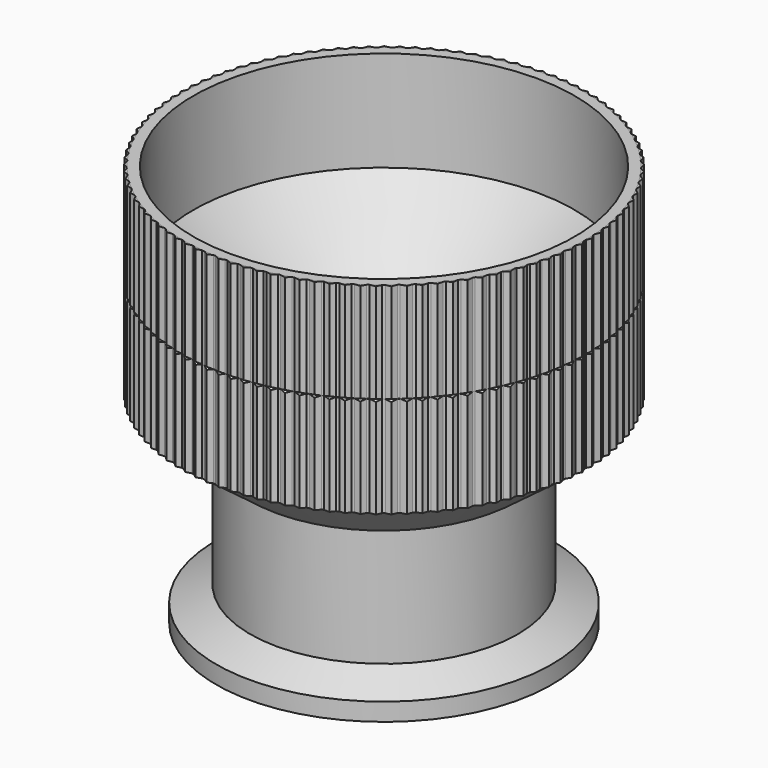
from build123d import *

# Parameters (mm, degrees)
F0_R      = 6
F1_DEPTH  = 6
F2_R      = 5.6
F3_DEPTH  = 3
F10_DEPTH = 31
F11_DEPTH = 25
F12_COUNT = 105


with BuildPart() as f1:
    # F0 (on Right) → F1 (new body)
    with BuildSketch(Plane.YZ):
        Circle(F0_R)
    extrude(amount=F1_DEPTH)

    # F2 (on face) → F3 (cut)
    with BuildSketch(Plane.YZ.offset(6)):
        Circle(F2_R)
    extrude(amount=-F3_DEPTH, mode=Mode.SUBTRACT)


with BuildPart() as f6:
    # F5 (on Right) → F6 (revolve)
    with BuildSketch(Plane.YZ):
        Polygon((6, 4.305355005), (6, 10.305355005), (5.6948992424, 10.305355005), (5.6948992424, 7.305355005), (3.011390429, 4.305355005), (3.011390429, 2.805355005), (3.011390429, -1.694644995), (5.011390429, -1.694644995), (5.011390429, -1.4897467336), (5.011390429, -1.1619703146), (4, -0.694644995), (4, 2.805355005), align=None)
    revolve(axis=Axis((0, 0, 5.6095318998), (0, 0, -1)))


with BuildPart() as f10:
    # F9 (on offset) → F10 (new body)
    with BuildSketch(Plane.XY.offset(35.305355005)):
        Polygon((-5.9907040559, -0.15034221), (-5.9907040559, 0.1501146035), (-6.068165414, 0), align=None)
    extrude(amount=-F10_DEPTH)

    # F11 (cut): a face of the model
    f11_faces = [f10.faces().sort_by_distance(p)[0] for p in [
        (-6.0165245086, -7.58688e-05, 35.305355005),
    ]]
    extrude(f11_faces, amount=-F11_DEPTH, mode=Mode.SUBTRACT)


with BuildPart() as f12_1:
    # F12: instance of F10
    add(f10.part.rotate(Axis((0, 0, 4.305355005), (0, 0, -1)), 1 * 360 / F12_COUNT))


with BuildPart() as f12_2:
    # F12: instance of F10
    add(f10.part.rotate(Axis((0, 0, 4.305355005), (0, 0, -1)), 2 * 360 / F12_COUNT))


with BuildPart() as f12_3:
    # F12: instance of F10
    add(f10.part.rotate(Axis((0, 0, 4.305355005), (0, 0, -1)), 3 * 360 / F12_COUNT))


with BuildPart() as f12_4:
    # F12: instance of F10
    add(f10.part.rotate(Axis((0, 0, 4.305355005), (0, 0, -1)), 4 * 360 / F12_COUNT))


with BuildPart() as f12_5:
    # F12: instance of F10
    add(f10.part.rotate(Axis((0, 0, 4.305355005), (0, 0, -1)), 5 * 360 / F12_COUNT))


with BuildPart() as f12_6:
    # F12: instance of F10
    add(f10.part.rotate(Axis((0, 0, 4.305355005), (0, 0, -1)), 6 * 360 / F12_COUNT))


with BuildPart() as f12_7:
    # F12: instance of F10
    add(f10.part.rotate(Axis((0, 0, 4.305355005), (0, 0, -1)), 7 * 360 / F12_COUNT))


with BuildPart() as f12_8:
    # F12: instance of F10
    add(f10.part.rotate(Axis((0, 0, 4.305355005), (0, 0, -1)), 8 * 360 / F12_COUNT))


with BuildPart() as f12_9:
    # F12: instance of F10
    add(f10.part.rotate(Axis((0, 0, 4.305355005), (0, 0, -1)), 9 * 360 / F12_COUNT))


with BuildPart() as f12_10:
    # F12: instance of F10
    add(f10.part.rotate(Axis((0, 0, 4.305355005), (0, 0, -1)), 10 * 360 / F12_COUNT))


with BuildPart() as f12_11:
    # F12: instance of F10
    add(f10.part.rotate(Axis((0, 0, 4.305355005), (0, 0, -1)), 11 * 360 / F12_COUNT))


with BuildPart() as f12_12:
    # F12: instance of F10
    add(f10.part.rotate(Axis((0, 0, 4.305355005), (0, 0, -1)), 12 * 360 / F12_COUNT))


with BuildPart() as f12_13:
    # F12: instance of F10
    add(f10.part.rotate(Axis((0, 0, 4.305355005), (0, 0, -1)), 13 * 360 / F12_COUNT))


with BuildPart() as f12_14:
    # F12: instance of F10
    add(f10.part.rotate(Axis((0, 0, 4.305355005), (0, 0, -1)), 14 * 360 / F12_COUNT))


with BuildPart() as f12_15:
    # F12: instance of F10
    add(f10.part.rotate(Axis((0, 0, 4.305355005), (0, 0, -1)), 15 * 360 / F12_COUNT))


with BuildPart() as f12_16:
    # F12: instance of F10
    add(f10.part.rotate(Axis((0, 0, 4.305355005), (0, 0, -1)), 16 * 360 / F12_COUNT))


with BuildPart() as f12_17:
    # F12: instance of F10
    add(f10.part.rotate(Axis((0, 0, 4.305355005), (0, 0, -1)), 17 * 360 / F12_COUNT))


with BuildPart() as f12_18:
    # F12: instance of F10
    add(f10.part.rotate(Axis((0, 0, 4.305355005), (0, 0, -1)), 18 * 360 / F12_COUNT))


with BuildPart() as f12_19:
    # F12: instance of F10
    add(f10.part.rotate(Axis((0, 0, 4.305355005), (0, 0, -1)), 19 * 360 / F12_COUNT))


with BuildPart() as f12_20:
    # F12: instance of F10
    add(f10.part.rotate(Axis((0, 0, 4.305355005), (0, 0, -1)), 20 * 360 / F12_COUNT))


with BuildPart() as f12_21:
    # F12: instance of F10
    add(f10.part.rotate(Axis((0, 0, 4.305355005), (0, 0, -1)), 21 * 360 / F12_COUNT))


with BuildPart() as f12_22:
    # F12: instance of F10
    add(f10.part.rotate(Axis((0, 0, 4.305355005), (0, 0, -1)), 22 * 360 / F12_COUNT))


with BuildPart() as f12_23:
    # F12: instance of F10
    add(f10.part.rotate(Axis((0, 0, 4.305355005), (0, 0, -1)), 23 * 360 / F12_COUNT))


with BuildPart() as f12_24:
    # F12: instance of F10
    add(f10.part.rotate(Axis((0, 0, 4.305355005), (0, 0, -1)), 24 * 360 / F12_COUNT))


with BuildPart() as f12_25:
    # F12: instance of F10
    add(f10.part.rotate(Axis((0, 0, 4.305355005), (0, 0, -1)), 25 * 360 / F12_COUNT))


with BuildPart() as f12_26:
    # F12: instance of F10
    add(f10.part.rotate(Axis((0, 0, 4.305355005), (0, 0, -1)), 26 * 360 / F12_COUNT))


with BuildPart() as f12_27:
    # F12: instance of F10
    add(f10.part.rotate(Axis((0, 0, 4.305355005), (0, 0, -1)), 27 * 360 / F12_COUNT))


with BuildPart() as f12_28:
    # F12: instance of F10
    add(f10.part.rotate(Axis((0, 0, 4.305355005), (0, 0, -1)), 28 * 360 / F12_COUNT))


with BuildPart() as f12_29:
    # F12: instance of F10
    add(f10.part.rotate(Axis((0, 0, 4.305355005), (0, 0, -1)), 29 * 360 / F12_COUNT))


with BuildPart() as f12_30:
    # F12: instance of F10
    add(f10.part.rotate(Axis((0, 0, 4.305355005), (0, 0, -1)), 30 * 360 / F12_COUNT))


with BuildPart() as f12_31:
    # F12: instance of F10
    add(f10.part.rotate(Axis((0, 0, 4.305355005), (0, 0, -1)), 31 * 360 / F12_COUNT))


with BuildPart() as f12_32:
    # F12: instance of F10
    add(f10.part.rotate(Axis((0, 0, 4.305355005), (0, 0, -1)), 32 * 360 / F12_COUNT))


with BuildPart() as f12_33:
    # F12: instance of F10
    add(f10.part.rotate(Axis((0, 0, 4.305355005), (0, 0, -1)), 33 * 360 / F12_COUNT))


with BuildPart() as f12_34:
    # F12: instance of F10
    add(f10.part.rotate(Axis((0, 0, 4.305355005), (0, 0, -1)), 34 * 360 / F12_COUNT))


with BuildPart() as f12_35:
    # F12: instance of F10
    add(f10.part.rotate(Axis((0, 0, 4.305355005), (0, 0, -1)), 35 * 360 / F12_COUNT))


with BuildPart() as f12_36:
    # F12: instance of F10
    add(f10.part.rotate(Axis((0, 0, 4.305355005), (0, 0, -1)), 36 * 360 / F12_COUNT))


with BuildPart() as f12_37:
    # F12: instance of F10
    add(f10.part.rotate(Axis((0, 0, 4.305355005), (0, 0, -1)), 37 * 360 / F12_COUNT))


with BuildPart() as f12_38:
    # F12: instance of F10
    add(f10.part.rotate(Axis((0, 0, 4.305355005), (0, 0, -1)), 38 * 360 / F12_COUNT))


with BuildPart() as f12_39:
    # F12: instance of F10
    add(f10.part.rotate(Axis((0, 0, 4.305355005), (0, 0, -1)), 39 * 360 / F12_COUNT))


with BuildPart() as f12_40:
    # F12: instance of F10
    add(f10.part.rotate(Axis((0, 0, 4.305355005), (0, 0, -1)), 40 * 360 / F12_COUNT))


with BuildPart() as f12_41:
    # F12: instance of F10
    add(f10.part.rotate(Axis((0, 0, 4.305355005), (0, 0, -1)), 41 * 360 / F12_COUNT))


with BuildPart() as f12_42:
    # F12: instance of F10
    add(f10.part.rotate(Axis((0, 0, 4.305355005), (0, 0, -1)), 42 * 360 / F12_COUNT))


with BuildPart() as f12_43:
    # F12: instance of F10
    add(f10.part.rotate(Axis((0, 0, 4.305355005), (0, 0, -1)), 43 * 360 / F12_COUNT))


with BuildPart() as f12_44:
    # F12: instance of F10
    add(f10.part.rotate(Axis((0, 0, 4.305355005), (0, 0, -1)), 44 * 360 / F12_COUNT))


with BuildPart() as f12_45:
    # F12: instance of F10
    add(f10.part.rotate(Axis((0, 0, 4.305355005), (0, 0, -1)), 45 * 360 / F12_COUNT))


with BuildPart() as f12_46:
    # F12: instance of F10
    add(f10.part.rotate(Axis((0, 0, 4.305355005), (0, 0, -1)), 46 * 360 / F12_COUNT))


with BuildPart() as f12_47:
    # F12: instance of F10
    add(f10.part.rotate(Axis((0, 0, 4.305355005), (0, 0, -1)), 47 * 360 / F12_COUNT))


with BuildPart() as f12_48:
    # F12: instance of F10
    add(f10.part.rotate(Axis((0, 0, 4.305355005), (0, 0, -1)), 48 * 360 / F12_COUNT))


with BuildPart() as f12_49:
    # F12: instance of F10
    add(f10.part.rotate(Axis((0, 0, 4.305355005), (0, 0, -1)), 49 * 360 / F12_COUNT))


with BuildPart() as f12_50:
    # F12: instance of F10
    add(f10.part.rotate(Axis((0, 0, 4.305355005), (0, 0, -1)), 50 * 360 / F12_COUNT))


with BuildPart() as f12_51:
    # F12: instance of F10
    add(f10.part.rotate(Axis((0, 0, 4.305355005), (0, 0, -1)), 51 * 360 / F12_COUNT))


with BuildPart() as f12_52:
    # F12: instance of F10
    add(f10.part.rotate(Axis((0, 0, 4.305355005), (0, 0, -1)), 52 * 360 / F12_COUNT))


with BuildPart() as f12_53:
    # F12: instance of F10
    add(f10.part.rotate(Axis((0, 0, 4.305355005), (0, 0, -1)), 53 * 360 / F12_COUNT))


with BuildPart() as f12_54:
    # F12: instance of F10
    add(f10.part.rotate(Axis((0, 0, 4.305355005), (0, 0, -1)), 54 * 360 / F12_COUNT))


with BuildPart() as f12_55:
    # F12: instance of F10
    add(f10.part.rotate(Axis((0, 0, 4.305355005), (0, 0, -1)), 55 * 360 / F12_COUNT))


with BuildPart() as f12_56:
    # F12: instance of F10
    add(f10.part.rotate(Axis((0, 0, 4.305355005), (0, 0, -1)), 56 * 360 / F12_COUNT))


with BuildPart() as f12_57:
    # F12: instance of F10
    add(f10.part.rotate(Axis((0, 0, 4.305355005), (0, 0, -1)), 57 * 360 / F12_COUNT))


with BuildPart() as f12_58:
    # F12: instance of F10
    add(f10.part.rotate(Axis((0, 0, 4.305355005), (0, 0, -1)), 58 * 360 / F12_COUNT))


with BuildPart() as f12_59:
    # F12: instance of F10
    add(f10.part.rotate(Axis((0, 0, 4.305355005), (0, 0, -1)), 59 * 360 / F12_COUNT))


with BuildPart() as f12_60:
    # F12: instance of F10
    add(f10.part.rotate(Axis((0, 0, 4.305355005), (0, 0, -1)), 60 * 360 / F12_COUNT))


with BuildPart() as f12_61:
    # F12: instance of F10
    add(f10.part.rotate(Axis((0, 0, 4.305355005), (0, 0, -1)), 61 * 360 / F12_COUNT))


with BuildPart() as f12_62:
    # F12: instance of F10
    add(f10.part.rotate(Axis((0, 0, 4.305355005), (0, 0, -1)), 62 * 360 / F12_COUNT))


with BuildPart() as f12_63:
    # F12: instance of F10
    add(f10.part.rotate(Axis((0, 0, 4.305355005), (0, 0, -1)), 63 * 360 / F12_COUNT))


with BuildPart() as f12_64:
    # F12: instance of F10
    add(f10.part.rotate(Axis((0, 0, 4.305355005), (0, 0, -1)), 64 * 360 / F12_COUNT))


with BuildPart() as f12_65:
    # F12: instance of F10
    add(f10.part.rotate(Axis((0, 0, 4.305355005), (0, 0, -1)), 65 * 360 / F12_COUNT))


with BuildPart() as f12_66:
    # F12: instance of F10
    add(f10.part.rotate(Axis((0, 0, 4.305355005), (0, 0, -1)), 66 * 360 / F12_COUNT))


with BuildPart() as f12_67:
    # F12: instance of F10
    add(f10.part.rotate(Axis((0, 0, 4.305355005), (0, 0, -1)), 67 * 360 / F12_COUNT))


with BuildPart() as f12_68:
    # F12: instance of F10
    add(f10.part.rotate(Axis((0, 0, 4.305355005), (0, 0, -1)), 68 * 360 / F12_COUNT))


with BuildPart() as f12_69:
    # F12: instance of F10
    add(f10.part.rotate(Axis((0, 0, 4.305355005), (0, 0, -1)), 69 * 360 / F12_COUNT))


with BuildPart() as f12_70:
    # F12: instance of F10
    add(f10.part.rotate(Axis((0, 0, 4.305355005), (0, 0, -1)), 70 * 360 / F12_COUNT))


with BuildPart() as f12_71:
    # F12: instance of F10
    add(f10.part.rotate(Axis((0, 0, 4.305355005), (0, 0, -1)), 71 * 360 / F12_COUNT))


with BuildPart() as f12_72:
    # F12: instance of F10
    add(f10.part.rotate(Axis((0, 0, 4.305355005), (0, 0, -1)), 72 * 360 / F12_COUNT))


with BuildPart() as f12_73:
    # F12: instance of F10
    add(f10.part.rotate(Axis((0, 0, 4.305355005), (0, 0, -1)), 73 * 360 / F12_COUNT))


with BuildPart() as f12_74:
    # F12: instance of F10
    add(f10.part.rotate(Axis((0, 0, 4.305355005), (0, 0, -1)), 74 * 360 / F12_COUNT))


with BuildPart() as f12_75:
    # F12: instance of F10
    add(f10.part.rotate(Axis((0, 0, 4.305355005), (0, 0, -1)), 75 * 360 / F12_COUNT))


with BuildPart() as f12_76:
    # F12: instance of F10
    add(f10.part.rotate(Axis((0, 0, 4.305355005), (0, 0, -1)), 76 * 360 / F12_COUNT))


with BuildPart() as f12_77:
    # F12: instance of F10
    add(f10.part.rotate(Axis((0, 0, 4.305355005), (0, 0, -1)), 77 * 360 / F12_COUNT))


with BuildPart() as f12_78:
    # F12: instance of F10
    add(f10.part.rotate(Axis((0, 0, 4.305355005), (0, 0, -1)), 78 * 360 / F12_COUNT))


with BuildPart() as f12_79:
    # F12: instance of F10
    add(f10.part.rotate(Axis((0, 0, 4.305355005), (0, 0, -1)), 79 * 360 / F12_COUNT))


with BuildPart() as f12_80:
    # F12: instance of F10
    add(f10.part.rotate(Axis((0, 0, 4.305355005), (0, 0, -1)), 80 * 360 / F12_COUNT))


with BuildPart() as f12_81:
    # F12: instance of F10
    add(f10.part.rotate(Axis((0, 0, 4.305355005), (0, 0, -1)), 81 * 360 / F12_COUNT))


with BuildPart() as f12_82:
    # F12: instance of F10
    add(f10.part.rotate(Axis((0, 0, 4.305355005), (0, 0, -1)), 82 * 360 / F12_COUNT))


with BuildPart() as f12_83:
    # F12: instance of F10
    add(f10.part.rotate(Axis((0, 0, 4.305355005), (0, 0, -1)), 83 * 360 / F12_COUNT))


with BuildPart() as f12_84:
    # F12: instance of F10
    add(f10.part.rotate(Axis((0, 0, 4.305355005), (0, 0, -1)), 84 * 360 / F12_COUNT))


with BuildPart() as f12_85:
    # F12: instance of F10
    add(f10.part.rotate(Axis((0, 0, 4.305355005), (0, 0, -1)), 85 * 360 / F12_COUNT))


with BuildPart() as f12_86:
    # F12: instance of F10
    add(f10.part.rotate(Axis((0, 0, 4.305355005), (0, 0, -1)), 86 * 360 / F12_COUNT))


with BuildPart() as f12_87:
    # F12: instance of F10
    add(f10.part.rotate(Axis((0, 0, 4.305355005), (0, 0, -1)), 87 * 360 / F12_COUNT))


with BuildPart() as f12_88:
    # F12: instance of F10
    add(f10.part.rotate(Axis((0, 0, 4.305355005), (0, 0, -1)), 88 * 360 / F12_COUNT))


with BuildPart() as f12_89:
    # F12: instance of F10
    add(f10.part.rotate(Axis((0, 0, 4.305355005), (0, 0, -1)), 89 * 360 / F12_COUNT))


with BuildPart() as f12_90:
    # F12: instance of F10
    add(f10.part.rotate(Axis((0, 0, 4.305355005), (0, 0, -1)), 90 * 360 / F12_COUNT))


with BuildPart() as f12_91:
    # F12: instance of F10
    add(f10.part.rotate(Axis((0, 0, 4.305355005), (0, 0, -1)), 91 * 360 / F12_COUNT))


with BuildPart() as f12_92:
    # F12: instance of F10
    add(f10.part.rotate(Axis((0, 0, 4.305355005), (0, 0, -1)), 92 * 360 / F12_COUNT))


with BuildPart() as f12_93:
    # F12: instance of F10
    add(f10.part.rotate(Axis((0, 0, 4.305355005), (0, 0, -1)), 93 * 360 / F12_COUNT))


with BuildPart() as f12_94:
    # F12: instance of F10
    add(f10.part.rotate(Axis((0, 0, 4.305355005), (0, 0, -1)), 94 * 360 / F12_COUNT))


with BuildPart() as f12_95:
    # F12: instance of F10
    add(f10.part.rotate(Axis((0, 0, 4.305355005), (0, 0, -1)), 95 * 360 / F12_COUNT))


with BuildPart() as f12_96:
    # F12: instance of F10
    add(f10.part.rotate(Axis((0, 0, 4.305355005), (0, 0, -1)), 96 * 360 / F12_COUNT))


with BuildPart() as f12_97:
    # F12: instance of F10
    add(f10.part.rotate(Axis((0, 0, 4.305355005), (0, 0, -1)), 97 * 360 / F12_COUNT))


with BuildPart() as f12_98:
    # F12: instance of F10
    add(f10.part.rotate(Axis((0, 0, 4.305355005), (0, 0, -1)), 98 * 360 / F12_COUNT))


with BuildPart() as f12_99:
    # F12: instance of F10
    add(f10.part.rotate(Axis((0, 0, 4.305355005), (0, 0, -1)), 99 * 360 / F12_COUNT))


with BuildPart() as f12_100:
    # F12: instance of F10
    add(f10.part.rotate(Axis((0, 0, 4.305355005), (0, 0, -1)), 100 * 360 / F12_COUNT))


with BuildPart() as f12_101:
    # F12: instance of F10
    add(f10.part.rotate(Axis((0, 0, 4.305355005), (0, 0, -1)), 101 * 360 / F12_COUNT))


with BuildPart() as f12_102:
    # F12: instance of F10
    add(f10.part.rotate(Axis((0, 0, 4.305355005), (0, 0, -1)), 102 * 360 / F12_COUNT))


with BuildPart() as f12_103:
    # F12: instance of F10
    add(f10.part.rotate(Axis((0, 0, 4.305355005), (0, 0, -1)), 103 * 360 / F12_COUNT))


with BuildPart() as f12_104:
    # F12: instance of F10
    add(f10.part.rotate(Axis((0, 0, 4.305355005), (0, 0, -1)), 104 * 360 / F12_COUNT))


with BuildPart() as f14_tool:
    # F13 (on Front) → F14 (revolve)
    with BuildSketch(Plane.XZ):
        Polygon((6.091067441, 7.3605600495), (5.9954494991, 7.305355005), (6.091067441, 7.2501499605), align=None)
    revolve(axis=Axis((0, 0, 6.7933266461), (0, 0, -1)))


with BuildPart() as f6_1:
    add(f6.part)

    # F14: cut by f14_tool
    add(f14_tool.part, mode=Mode.SUBTRACT)


with BuildPart() as f10_1:
    add(f10.part)

    # F14: cut by f14_tool
    add(f14_tool.part, mode=Mode.SUBTRACT)


with BuildPart() as f12_1_1:
    add(f12_1.part)

    # F14: cut by f14_tool
    add(f14_tool.part, mode=Mode.SUBTRACT)


with BuildPart() as f12_2_1:
    add(f12_2.part)

    # F14: cut by f14_tool
    add(f14_tool.part, mode=Mode.SUBTRACT)


with BuildPart() as f12_3_1:
    add(f12_3.part)

    # F14: cut by f14_tool
    add(f14_tool.part, mode=Mode.SUBTRACT)


with BuildPart() as f12_4_1:
    add(f12_4.part)

    # F14: cut by f14_tool
    add(f14_tool.part, mode=Mode.SUBTRACT)


with BuildPart() as f12_5_1:
    add(f12_5.part)

    # F14: cut by f14_tool
    add(f14_tool.part, mode=Mode.SUBTRACT)


with BuildPart() as f12_6_1:
    add(f12_6.part)

    # F14: cut by f14_tool
    add(f14_tool.part, mode=Mode.SUBTRACT)


with BuildPart() as f12_7_1:
    add(f12_7.part)

    # F14: cut by f14_tool
    add(f14_tool.part, mode=Mode.SUBTRACT)


with BuildPart() as f12_8_1:
    add(f12_8.part)

    # F14: cut by f14_tool
    add(f14_tool.part, mode=Mode.SUBTRACT)


with BuildPart() as f12_9_1:
    add(f12_9.part)

    # F14: cut by f14_tool
    add(f14_tool.part, mode=Mode.SUBTRACT)


with BuildPart() as f12_10_1:
    add(f12_10.part)

    # F14: cut by f14_tool
    add(f14_tool.part, mode=Mode.SUBTRACT)


with BuildPart() as f12_11_1:
    add(f12_11.part)

    # F14: cut by f14_tool
    add(f14_tool.part, mode=Mode.SUBTRACT)


with BuildPart() as f12_12_1:
    add(f12_12.part)

    # F14: cut by f14_tool
    add(f14_tool.part, mode=Mode.SUBTRACT)


with BuildPart() as f12_13_1:
    add(f12_13.part)

    # F14: cut by f14_tool
    add(f14_tool.part, mode=Mode.SUBTRACT)


with BuildPart() as f12_14_1:
    add(f12_14.part)

    # F14: cut by f14_tool
    add(f14_tool.part, mode=Mode.SUBTRACT)


with BuildPart() as f12_15_1:
    add(f12_15.part)

    # F14: cut by f14_tool
    add(f14_tool.part, mode=Mode.SUBTRACT)


with BuildPart() as f12_16_1:
    add(f12_16.part)

    # F14: cut by f14_tool
    add(f14_tool.part, mode=Mode.SUBTRACT)


with BuildPart() as f12_17_1:
    add(f12_17.part)

    # F14: cut by f14_tool
    add(f14_tool.part, mode=Mode.SUBTRACT)


with BuildPart() as f12_18_1:
    add(f12_18.part)

    # F14: cut by f14_tool
    add(f14_tool.part, mode=Mode.SUBTRACT)


with BuildPart() as f12_19_1:
    add(f12_19.part)

    # F14: cut by f14_tool
    add(f14_tool.part, mode=Mode.SUBTRACT)


with BuildPart() as f12_20_1:
    add(f12_20.part)

    # F14: cut by f14_tool
    add(f14_tool.part, mode=Mode.SUBTRACT)


with BuildPart() as f12_21_1:
    add(f12_21.part)

    # F14: cut by f14_tool
    add(f14_tool.part, mode=Mode.SUBTRACT)


with BuildPart() as f12_22_1:
    add(f12_22.part)

    # F14: cut by f14_tool
    add(f14_tool.part, mode=Mode.SUBTRACT)


with BuildPart() as f12_23_1:
    add(f12_23.part)

    # F14: cut by f14_tool
    add(f14_tool.part, mode=Mode.SUBTRACT)


with BuildPart() as f12_24_1:
    add(f12_24.part)

    # F14: cut by f14_tool
    add(f14_tool.part, mode=Mode.SUBTRACT)


with BuildPart() as f12_25_1:
    add(f12_25.part)

    # F14: cut by f14_tool
    add(f14_tool.part, mode=Mode.SUBTRACT)


with BuildPart() as f12_26_1:
    add(f12_26.part)

    # F14: cut by f14_tool
    add(f14_tool.part, mode=Mode.SUBTRACT)


with BuildPart() as f12_27_1:
    add(f12_27.part)

    # F14: cut by f14_tool
    add(f14_tool.part, mode=Mode.SUBTRACT)


with BuildPart() as f12_28_1:
    add(f12_28.part)

    # F14: cut by f14_tool
    add(f14_tool.part, mode=Mode.SUBTRACT)


with BuildPart() as f12_29_1:
    add(f12_29.part)

    # F14: cut by f14_tool
    add(f14_tool.part, mode=Mode.SUBTRACT)


with BuildPart() as f12_30_1:
    add(f12_30.part)

    # F14: cut by f14_tool
    add(f14_tool.part, mode=Mode.SUBTRACT)


with BuildPart() as f12_31_1:
    add(f12_31.part)

    # F14: cut by f14_tool
    add(f14_tool.part, mode=Mode.SUBTRACT)


with BuildPart() as f12_32_1:
    add(f12_32.part)

    # F14: cut by f14_tool
    add(f14_tool.part, mode=Mode.SUBTRACT)


with BuildPart() as f12_33_1:
    add(f12_33.part)

    # F14: cut by f14_tool
    add(f14_tool.part, mode=Mode.SUBTRACT)


with BuildPart() as f12_34_1:
    add(f12_34.part)

    # F14: cut by f14_tool
    add(f14_tool.part, mode=Mode.SUBTRACT)


with BuildPart() as f12_35_1:
    add(f12_35.part)

    # F14: cut by f14_tool
    add(f14_tool.part, mode=Mode.SUBTRACT)


with BuildPart() as f12_36_1:
    add(f12_36.part)

    # F14: cut by f14_tool
    add(f14_tool.part, mode=Mode.SUBTRACT)


with BuildPart() as f12_37_1:
    add(f12_37.part)

    # F14: cut by f14_tool
    add(f14_tool.part, mode=Mode.SUBTRACT)


with BuildPart() as f12_38_1:
    add(f12_38.part)

    # F14: cut by f14_tool
    add(f14_tool.part, mode=Mode.SUBTRACT)


with BuildPart() as f12_39_1:
    add(f12_39.part)

    # F14: cut by f14_tool
    add(f14_tool.part, mode=Mode.SUBTRACT)


with BuildPart() as f12_40_1:
    add(f12_40.part)

    # F14: cut by f14_tool
    add(f14_tool.part, mode=Mode.SUBTRACT)


with BuildPart() as f12_41_1:
    add(f12_41.part)

    # F14: cut by f14_tool
    add(f14_tool.part, mode=Mode.SUBTRACT)


with BuildPart() as f12_42_1:
    add(f12_42.part)

    # F14: cut by f14_tool
    add(f14_tool.part, mode=Mode.SUBTRACT)


with BuildPart() as f12_43_1:
    add(f12_43.part)

    # F14: cut by f14_tool
    add(f14_tool.part, mode=Mode.SUBTRACT)


with BuildPart() as f12_44_1:
    add(f12_44.part)

    # F14: cut by f14_tool
    add(f14_tool.part, mode=Mode.SUBTRACT)


with BuildPart() as f12_45_1:
    add(f12_45.part)

    # F14: cut by f14_tool
    add(f14_tool.part, mode=Mode.SUBTRACT)


with BuildPart() as f12_46_1:
    add(f12_46.part)

    # F14: cut by f14_tool
    add(f14_tool.part, mode=Mode.SUBTRACT)


with BuildPart() as f12_47_1:
    add(f12_47.part)

    # F14: cut by f14_tool
    add(f14_tool.part, mode=Mode.SUBTRACT)


with BuildPart() as f12_48_1:
    add(f12_48.part)

    # F14: cut by f14_tool
    add(f14_tool.part, mode=Mode.SUBTRACT)


with BuildPart() as f12_49_1:
    add(f12_49.part)

    # F14: cut by f14_tool
    add(f14_tool.part, mode=Mode.SUBTRACT)


with BuildPart() as f12_50_1:
    add(f12_50.part)

    # F14: cut by f14_tool
    add(f14_tool.part, mode=Mode.SUBTRACT)


with BuildPart() as f12_51_1:
    add(f12_51.part)

    # F14: cut by f14_tool
    add(f14_tool.part, mode=Mode.SUBTRACT)


with BuildPart() as f12_52_1:
    add(f12_52.part)

    # F14: cut by f14_tool
    add(f14_tool.part, mode=Mode.SUBTRACT)


with BuildPart() as f12_53_1:
    add(f12_53.part)

    # F14: cut by f14_tool
    add(f14_tool.part, mode=Mode.SUBTRACT)


with BuildPart() as f12_54_1:
    add(f12_54.part)

    # F14: cut by f14_tool
    add(f14_tool.part, mode=Mode.SUBTRACT)


with BuildPart() as f12_55_1:
    add(f12_55.part)

    # F14: cut by f14_tool
    add(f14_tool.part, mode=Mode.SUBTRACT)


with BuildPart() as f12_56_1:
    add(f12_56.part)

    # F14: cut by f14_tool
    add(f14_tool.part, mode=Mode.SUBTRACT)


with BuildPart() as f12_57_1:
    add(f12_57.part)

    # F14: cut by f14_tool
    add(f14_tool.part, mode=Mode.SUBTRACT)


with BuildPart() as f12_58_1:
    add(f12_58.part)

    # F14: cut by f14_tool
    add(f14_tool.part, mode=Mode.SUBTRACT)


with BuildPart() as f12_59_1:
    add(f12_59.part)

    # F14: cut by f14_tool
    add(f14_tool.part, mode=Mode.SUBTRACT)


with BuildPart() as f12_60_1:
    add(f12_60.part)

    # F14: cut by f14_tool
    add(f14_tool.part, mode=Mode.SUBTRACT)


with BuildPart() as f12_61_1:
    add(f12_61.part)

    # F14: cut by f14_tool
    add(f14_tool.part, mode=Mode.SUBTRACT)


with BuildPart() as f12_62_1:
    add(f12_62.part)

    # F14: cut by f14_tool
    add(f14_tool.part, mode=Mode.SUBTRACT)


with BuildPart() as f12_63_1:
    add(f12_63.part)

    # F14: cut by f14_tool
    add(f14_tool.part, mode=Mode.SUBTRACT)


with BuildPart() as f12_64_1:
    add(f12_64.part)

    # F14: cut by f14_tool
    add(f14_tool.part, mode=Mode.SUBTRACT)


with BuildPart() as f12_65_1:
    add(f12_65.part)

    # F14: cut by f14_tool
    add(f14_tool.part, mode=Mode.SUBTRACT)


with BuildPart() as f12_66_1:
    add(f12_66.part)

    # F14: cut by f14_tool
    add(f14_tool.part, mode=Mode.SUBTRACT)


with BuildPart() as f12_67_1:
    add(f12_67.part)

    # F14: cut by f14_tool
    add(f14_tool.part, mode=Mode.SUBTRACT)


with BuildPart() as f12_68_1:
    add(f12_68.part)

    # F14: cut by f14_tool
    add(f14_tool.part, mode=Mode.SUBTRACT)


with BuildPart() as f12_69_1:
    add(f12_69.part)

    # F14: cut by f14_tool
    add(f14_tool.part, mode=Mode.SUBTRACT)


with BuildPart() as f12_70_1:
    add(f12_70.part)

    # F14: cut by f14_tool
    add(f14_tool.part, mode=Mode.SUBTRACT)


with BuildPart() as f12_71_1:
    add(f12_71.part)

    # F14: cut by f14_tool
    add(f14_tool.part, mode=Mode.SUBTRACT)


with BuildPart() as f12_72_1:
    add(f12_72.part)

    # F14: cut by f14_tool
    add(f14_tool.part, mode=Mode.SUBTRACT)


with BuildPart() as f12_73_1:
    add(f12_73.part)

    # F14: cut by f14_tool
    add(f14_tool.part, mode=Mode.SUBTRACT)


with BuildPart() as f12_74_1:
    add(f12_74.part)

    # F14: cut by f14_tool
    add(f14_tool.part, mode=Mode.SUBTRACT)


with BuildPart() as f12_75_1:
    add(f12_75.part)

    # F14: cut by f14_tool
    add(f14_tool.part, mode=Mode.SUBTRACT)


with BuildPart() as f12_76_1:
    add(f12_76.part)

    # F14: cut by f14_tool
    add(f14_tool.part, mode=Mode.SUBTRACT)


with BuildPart() as f12_77_1:
    add(f12_77.part)

    # F14: cut by f14_tool
    add(f14_tool.part, mode=Mode.SUBTRACT)


with BuildPart() as f12_78_1:
    add(f12_78.part)

    # F14: cut by f14_tool
    add(f14_tool.part, mode=Mode.SUBTRACT)


with BuildPart() as f12_79_1:
    add(f12_79.part)

    # F14: cut by f14_tool
    add(f14_tool.part, mode=Mode.SUBTRACT)


with BuildPart() as f12_80_1:
    add(f12_80.part)

    # F14: cut by f14_tool
    add(f14_tool.part, mode=Mode.SUBTRACT)


with BuildPart() as f12_81_1:
    add(f12_81.part)

    # F14: cut by f14_tool
    add(f14_tool.part, mode=Mode.SUBTRACT)


with BuildPart() as f12_82_1:
    add(f12_82.part)

    # F14: cut by f14_tool
    add(f14_tool.part, mode=Mode.SUBTRACT)


with BuildPart() as f12_83_1:
    add(f12_83.part)

    # F14: cut by f14_tool
    add(f14_tool.part, mode=Mode.SUBTRACT)


with BuildPart() as f12_84_1:
    add(f12_84.part)

    # F14: cut by f14_tool
    add(f14_tool.part, mode=Mode.SUBTRACT)


with BuildPart() as f12_85_1:
    add(f12_85.part)

    # F14: cut by f14_tool
    add(f14_tool.part, mode=Mode.SUBTRACT)


with BuildPart() as f12_86_1:
    add(f12_86.part)

    # F14: cut by f14_tool
    add(f14_tool.part, mode=Mode.SUBTRACT)


with BuildPart() as f12_87_1:
    add(f12_87.part)

    # F14: cut by f14_tool
    add(f14_tool.part, mode=Mode.SUBTRACT)


with BuildPart() as f12_88_1:
    add(f12_88.part)

    # F14: cut by f14_tool
    add(f14_tool.part, mode=Mode.SUBTRACT)


with BuildPart() as f12_89_1:
    add(f12_89.part)

    # F14: cut by f14_tool
    add(f14_tool.part, mode=Mode.SUBTRACT)


with BuildPart() as f12_90_1:
    add(f12_90.part)

    # F14: cut by f14_tool
    add(f14_tool.part, mode=Mode.SUBTRACT)


with BuildPart() as f12_91_1:
    add(f12_91.part)

    # F14: cut by f14_tool
    add(f14_tool.part, mode=Mode.SUBTRACT)


with BuildPart() as f12_92_1:
    add(f12_92.part)

    # F14: cut by f14_tool
    add(f14_tool.part, mode=Mode.SUBTRACT)


with BuildPart() as f12_93_1:
    add(f12_93.part)

    # F14: cut by f14_tool
    add(f14_tool.part, mode=Mode.SUBTRACT)


with BuildPart() as f12_94_1:
    add(f12_94.part)

    # F14: cut by f14_tool
    add(f14_tool.part, mode=Mode.SUBTRACT)


with BuildPart() as f12_95_1:
    add(f12_95.part)

    # F14: cut by f14_tool
    add(f14_tool.part, mode=Mode.SUBTRACT)


with BuildPart() as f12_96_1:
    add(f12_96.part)

    # F14: cut by f14_tool
    add(f14_tool.part, mode=Mode.SUBTRACT)


with BuildPart() as f12_97_1:
    add(f12_97.part)

    # F14: cut by f14_tool
    add(f14_tool.part, mode=Mode.SUBTRACT)


with BuildPart() as f12_98_1:
    add(f12_98.part)

    # F14: cut by f14_tool
    add(f14_tool.part, mode=Mode.SUBTRACT)


with BuildPart() as f12_99_1:
    add(f12_99.part)

    # F14: cut by f14_tool
    add(f14_tool.part, mode=Mode.SUBTRACT)


with BuildPart() as f12_100_1:
    add(f12_100.part)

    # F14: cut by f14_tool
    add(f14_tool.part, mode=Mode.SUBTRACT)


with BuildPart() as f12_101_1:
    add(f12_101.part)

    # F14: cut by f14_tool
    add(f14_tool.part, mode=Mode.SUBTRACT)


with BuildPart() as f12_102_1:
    add(f12_102.part)

    # F14: cut by f14_tool
    add(f14_tool.part, mode=Mode.SUBTRACT)


with BuildPart() as f12_103_1:
    add(f12_103.part)

    # F14: cut by f14_tool
    add(f14_tool.part, mode=Mode.SUBTRACT)


with BuildPart() as f12_104_1:
    add(f12_104.part)

    # F14: cut by f14_tool
    add(f14_tool.part, mode=Mode.SUBTRACT)


solid = Compound([f6_1.part, f10_1.part, f12_1_1.part, f12_2_1.part, f12_3_1.part, f12_4_1.part, f12_5_1.part, f12_6_1.part, f12_7_1.part, f12_8_1.part, f12_9_1.part, f12_10_1.part, f12_11_1.part, f12_12_1.part, f12_13_1.part, f12_14_1.part, f12_15_1.part, f12_16_1.part, f12_17_1.part, f12_18_1.part, f12_19_1.part, f12_20_1.part, f12_21_1.part, f12_22_1.part, f12_23_1.part, f12_24_1.part, f12_25_1.part, f12_26_1.part, f12_27_1.part, f12_28_1.part, f12_29_1.part, f12_30_1.part, f12_31_1.part, f12_32_1.part, f12_33_1.part, f12_34_1.part, f12_35_1.part, f12_36_1.part, f12_37_1.part, f12_38_1.part, f12_39_1.part, f12_40_1.part, f12_41_1.part, f12_42_1.part, f12_43_1.part, f12_44_1.part, f12_45_1.part, f12_46_1.part, f12_47_1.part, f12_48_1.part, f12_49_1.part, f12_50_1.part, f12_51_1.part, f12_52_1.part, f12_53_1.part, f12_54_1.part, f12_55_1.part, f12_56_1.part, f12_57_1.part, f12_58_1.part, f12_59_1.part, f12_60_1.part, f12_61_1.part, f12_62_1.part, f12_63_1.part, f12_64_1.part, f12_65_1.part, f12_66_1.part, f12_67_1.part, f12_68_1.part, f12_69_1.part, f12_70_1.part, f12_71_1.part, f12_72_1.part, f12_73_1.part, f12_74_1.part, f12_75_1.part, f12_76_1.part, f12_77_1.part, f12_78_1.part, f12_79_1.part, f12_80_1.part, f12_81_1.part, f12_82_1.part, f12_83_1.part, f12_84_1.part, f12_85_1.part, f12_86_1.part, f12_87_1.part, f12_88_1.part, f12_89_1.part, f12_90_1.part, f12_91_1.part, f12_92_1.part, f12_93_1.part, f12_94_1.part, f12_95_1.part, f12_96_1.part, f12_97_1.part, f12_98_1.part, f12_99_1.part, f12_100_1.part, f12_101_1.part, f12_102_1.part, f12_103_1.part, f12_104_1.part])
